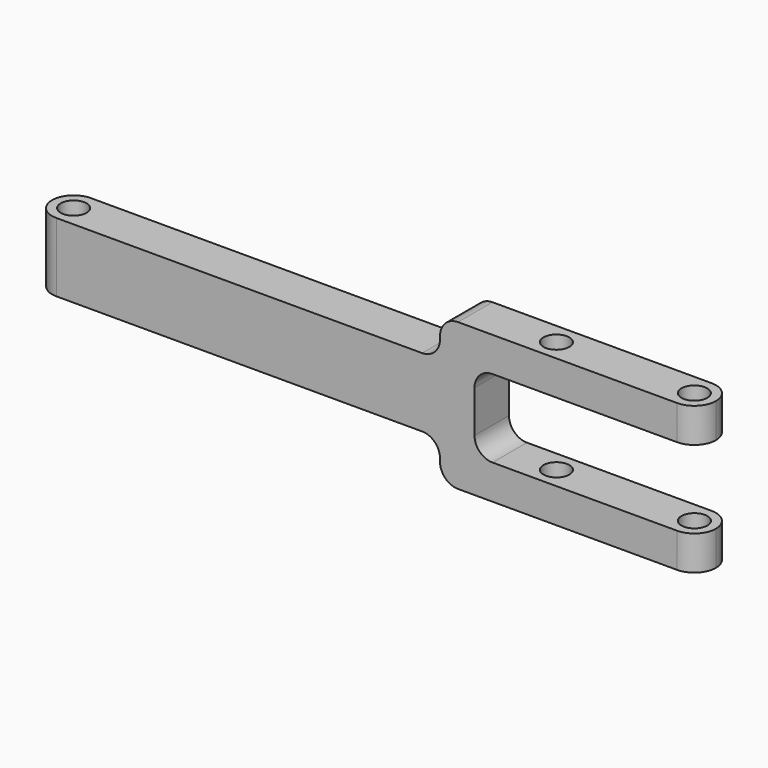
from build123d import *

# Parameters (mm, degrees)
F1_DEPTH = 54.102
F2_D     = 9.525
F3_W     = 74.6125
F3_H     = 28.702
F3_W_2   = 36.2260771513
F4_W     = 161.925
F4_H     = 27.051
F5_DEPTH = 25.4
F7_R     = 6.604


# Not quite as in the source:
# - a pattern or mirror of a feature is missing from the dataset's text; its kind, count and spacing are read off the source's solid


with BuildPart() as f1:
    # F0 (on Top) → F1 (new body)
    with BuildSketch(Plane.XY):
        with BuildLine():
            ThreePointArc((236.5375, -7.9375), (234.2126600757, -2.3248399243), (228.6, 0))
            Line((228.6, 0), (228.6, -15.875))
            ThreePointArc((228.6, -15.875), (234.2126600757, -13.5501600757), (236.5375, -7.9375))
        make_face()
        with BuildLine():
            Line((228.6, -15.875), (228.6, 0))
            ThreePointArc((228.6, 0), (220.6625, -7.9375), (228.6, -15.875))
        make_face()
        with BuildLine():
            Line((228.6, 0), (0, 0))
            ThreePointArc((0, 0), (5.6126600757, -2.3248399243), (7.9375, -7.9375))
            ThreePointArc((7.9375, -7.9375), (5.6126600757, -13.5501600757), (0, -15.875))
            Line((0, -15.875), (228.6, -15.875))
            ThreePointArc((228.6, -15.875), (220.6625, -7.9375), (228.6, 0))
        make_face()
        with BuildLine():
            ThreePointArc((7.9375, -7.9375), (5.6126600757, -2.3248399243), (0, 0))
            Line((0, 0), (0, -15.875))
            ThreePointArc((0, -15.875), (5.6126600757, -13.5501600757), (7.9375, -7.9375))
        make_face()
        with BuildLine():
            Line((0, -15.875), (0, 0))
            ThreePointArc((0, 0), (-7.9375, -7.9375), (0, -15.875))
        make_face()
    extrude(amount=F1_DEPTH)

    # F2 (through all)
    with Locations(Plane(origin=(0, 0, 0), x_dir=(1, 0, 0), z_dir=(0, 0, -1))):
        with Locations((0, 7.9375), (177.8, 7.9375), (228.6, 7.9375)):
            Hole(F2_D / 2)

    # F3 (on Front) + F4 (on Front) → F5 (cut)
    with BuildSketch(Plane.XZ):
        with Locations((191.29375, 27.051)):
            Rectangle(F3_W, F3_H)
        with Locations((246.7130385756, 27.051)):
            Rectangle(F3_W_2, F3_H)
    with BuildSketch(Plane.XZ):
        with Locations((60.325, 53.2765)):
            Rectangle(F4_W, F4_H)
    f5 = extrude(amount=F5_DEPTH, mode=Mode.SUBTRACT)

    # F5_copies: F5 across plane
    add(f5.mirror(Plane(origin=(0, 0, 27.051), x_dir=(-1, 0, 0), z_dir=(0, 0, -1))), mode=Mode.SUBTRACT)

    # F7
    f7_edges = [f1.edges().sort_by_distance(p)[0] for p in [
        (141.2875, -7.9375, 39.751),
        (141.2875, -7.9375, 54.102),
        (153.9875, -7.9375, 12.7),
        (153.9875, -7.9375, 41.402),
        (141.2875, -7.9375, 0),
        (141.2875, -7.9375, 14.351),
    ]]
    fillet(f7_edges, radius=F7_R)


solid = f1.part
